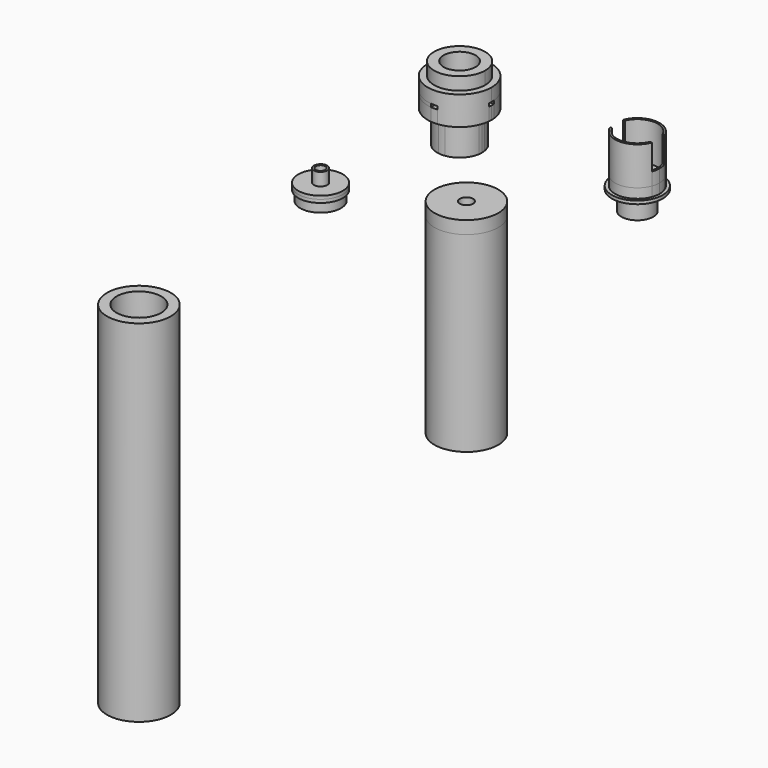
from build123d import *
from build123d import SkipClean  # not in build123d's __all__

# Parameters (mm, degrees)
F1_DEPTH  = 2
F2_DEPTH  = 7
F3_DEPTH  = 0.5
F5_DEPTH  = 2
F4_R      = 2.5
F6_DEPTH  = 4
F7_DEPTH  = 1
F8_R      = 2.5
F8_R_2    = 0.75
F9_DEPTH  = 2
F10_DEPTH = 5
F11_DEPTH = 2
F12_DEPTH = 6
F13_R     = 3.5
F13_R_2   = 3.2
F13_R_3   = 2.9
F14_DEPTH = 0.5
F15_DEPTH = 2
F13_R_4   = 1.05
F16_DEPTH = 0.5
F13_R_5   = 0.75
F17_DEPTH = 2.5
F18_R     = 5
F18_R_2   = 4
F19_DEPTH = 30
F18_R_3   = 1.35
F18_R_4   = 1.05
F20_DEPTH = 23
F21_DEPTH = 2
F22_R     = 4
F22_R_2   = 3.5
F23_DEPTH = 0.5
F24_R     = 5
F24_R_2   = 3.5
F25_DEPTH = 55
F26_DEPTH = 5


with BuildPart() as f1:
    # F0 (on Top) → F1 (new body)
    with BuildSketch(Plane.XY):
        with BuildLine():
            Line((-52.3957748821, 53.1159022585), (-50.8849393117, 53.1159022585))
            ThreePointArc((-50.8849393117, 53.1159022585), (-52.3243425913, 56.1514361644), (-55.3598764972, 57.590839444))
            Line((-55.3598764972, 57.590839444), (-55.3598764972, 56.0800038736))
            ThreePointArc((-55.3598764972, 56.0800038736), (-53.3850027631, 55.0907759926), (-52.3957748821, 53.1159022585))
        make_face()
        with BuildLine():
            Line((-59.3239781124, 53.1159022585), (-60.8348136828, 53.1159022585))
            ThreePointArc((-60.8348136828, 53.1159022585), (-60.8598764972, 52.6159022585), (-60.8348136828, 52.1159022585))
            Line((-60.8348136828, 52.1159022585), (-59.3239781124, 52.1159022585))
            ThreePointArc((-59.3239781124, 52.1159022585), (-59.3598764972, 52.6159022585), (-59.3239781124, 53.1159022585))
        make_face()
        with BuildLine():
            ThreePointArc((-56.3598764972, 47.6409650729), (-55.8598764972, 47.6159022585), (-55.3598764972, 47.6409650729))
            Line((-55.3598764972, 47.6409650729), (-55.3598764972, 49.1518006433))
            ThreePointArc((-55.3598764972, 49.1518006433), (-55.8598764972, 49.1159022585), (-56.3598764972, 49.1518006433))
            Line((-56.3598764972, 49.1518006433), (-56.3598764972, 47.6409650729))
        make_face()
        with BuildLine():
            ThreePointArc((-55.3598764972, 47.6409650729), (-52.3243425913, 49.0803683525), (-50.8849393117, 52.1159022585))
            Line((-50.8849393117, 52.1159022585), (-52.3957748821, 52.1159022585))
            ThreePointArc((-52.3957748821, 52.1159022585), (-53.3850027631, 50.1410285243), (-55.3598764972, 49.1518006433))
            Line((-55.3598764972, 49.1518006433), (-55.3598764972, 47.6409650729))
        make_face()
        with BuildLine():
            ThreePointArc((-52.3598764972, 52.6159022585), (-52.3688626292, 52.8665457773), (-52.3957748821, 53.1159022585))
            ThreePointArc((-52.3957748821, 53.1159022585), (-53.3850027631, 55.0907759926), (-55.3598764972, 56.0800038736))
            ThreePointArc((-55.3598764972, 56.0800038736), (-55.8598764972, 56.1159022585), (-56.3598764972, 56.0800038736))
            ThreePointArc((-56.3598764972, 56.0800038736), (-58.3347502314, 55.0907759926), (-59.3239781124, 53.1159022585))
            ThreePointArc((-59.3239781124, 53.1159022585), (-59.3598764972, 52.6159022585), (-59.3239781124, 52.1159022585))
            ThreePointArc((-59.3239781124, 52.1159022585), (-58.3347502314, 50.1410285243), (-56.3598764972, 49.1518006433))
            ThreePointArc((-56.3598764972, 49.1518006433), (-55.8598764972, 49.1159022585), (-55.3598764972, 49.1518006433))
            ThreePointArc((-55.3598764972, 49.1518006433), (-53.3850027631, 50.1410285243), (-52.3957748821, 52.1159022585))
            ThreePointArc((-52.3957748821, 52.1159022585), (-52.3688626292, 52.3652587397), (-52.3598764972, 52.6159022585))
        make_face()
        with BuildLine():
            ThreePointArc((-50.8849393117, 52.1159022585), (-50.8661461317, 52.3655883832), (-50.8598764972, 52.6159022585))
            ThreePointArc((-50.8598764972, 52.6159022585), (-50.8661461317, 52.8662161338), (-50.8849393117, 53.1159022585))
            Line((-50.8849393117, 53.1159022585), (-52.3957748821, 53.1159022585))
            ThreePointArc((-52.3957748821, 53.1159022585), (-52.3688626292, 52.8665457773), (-52.3598764972, 52.6159022585))
            ThreePointArc((-52.3598764972, 52.6159022585), (-52.3688626292, 52.3652587397), (-52.3957748821, 52.1159022585))
            Line((-52.3957748821, 52.1159022585), (-50.8849393117, 52.1159022585))
        make_face()
        with BuildLine():
            ThreePointArc((-60.8348136828, 52.1159022585), (-59.3954104032, 49.0803683525), (-56.3598764972, 47.6409650729))
            Line((-56.3598764972, 47.6409650729), (-56.3598764972, 49.1518006433))
            ThreePointArc((-56.3598764972, 49.1518006433), (-58.3347502314, 50.1410285243), (-59.3239781124, 52.1159022585))
            Line((-59.3239781124, 52.1159022585), (-60.8348136828, 52.1159022585))
        make_face()
        with BuildLine():
            Line((-55.3598764972, 56.0800038736), (-55.3598764972, 57.590839444))
            ThreePointArc((-55.3598764972, 57.590839444), (-55.8598764972, 57.6159022585), (-56.3598764972, 57.590839444))
            Line((-56.3598764972, 57.590839444), (-56.3598764972, 56.0800038736))
            ThreePointArc((-56.3598764972, 56.0800038736), (-55.8598764972, 56.1159022585), (-55.3598764972, 56.0800038736))
        make_face()
        with BuildLine():
            Line((-56.3598764972, 56.0800038736), (-56.3598764972, 57.590839444))
            ThreePointArc((-56.3598764972, 57.590839444), (-59.3954104032, 56.1514361644), (-60.8348136828, 53.1159022585))
            Line((-60.8348136828, 53.1159022585), (-59.3239781124, 53.1159022585))
            ThreePointArc((-59.3239781124, 53.1159022585), (-58.3347502314, 55.0907759926), (-56.3598764972, 56.0800038736))
        make_face()
    extrude(amount=-F1_DEPTH)

    # F0 (on Top) → F2 (join)
    with BuildSketch(Plane.XY):
        with BuildLine():
            ThreePointArc((-52.3598764972, 52.6159022585), (-52.3688626292, 52.8665457773), (-52.3957748821, 53.1159022585))
            ThreePointArc((-52.3957748821, 53.1159022585), (-53.3850027631, 55.0907759926), (-55.3598764972, 56.0800038736))
            ThreePointArc((-55.3598764972, 56.0800038736), (-55.8598764972, 56.1159022585), (-56.3598764972, 56.0800038736))
            ThreePointArc((-56.3598764972, 56.0800038736), (-58.3347502314, 55.0907759926), (-59.3239781124, 53.1159022585))
            ThreePointArc((-59.3239781124, 53.1159022585), (-59.3598764972, 52.6159022585), (-59.3239781124, 52.1159022585))
            ThreePointArc((-59.3239781124, 52.1159022585), (-58.3347502314, 50.1410285243), (-56.3598764972, 49.1518006433))
            ThreePointArc((-56.3598764972, 49.1518006433), (-55.8598764972, 49.1159022585), (-55.3598764972, 49.1518006433))
            ThreePointArc((-55.3598764972, 49.1518006433), (-53.3850027631, 50.1410285243), (-52.3957748821, 52.1159022585))
            ThreePointArc((-52.3957748821, 52.1159022585), (-52.3688626292, 52.3652587397), (-52.3598764972, 52.6159022585))
        make_face()
    extrude(amount=-F2_DEPTH)

    # F0 (on Top) → F3 (join)
    with BuildSketch(Plane.XY):
        with BuildLine():
            Line((-52.3957748821, 53.1159022585), (-50.8849393117, 53.1159022585))
            ThreePointArc((-50.8849393117, 53.1159022585), (-52.3243425913, 56.1514361644), (-55.3598764972, 57.590839444))
            Line((-55.3598764972, 57.590839444), (-55.3598764972, 56.0800038736))
            ThreePointArc((-55.3598764972, 56.0800038736), (-53.3850027631, 55.0907759926), (-52.3957748821, 53.1159022585))
        make_face()
        with BuildLine():
            ThreePointArc((-55.3598764972, 47.6409650729), (-52.3243425913, 49.0803683525), (-50.8849393117, 52.1159022585))
            Line((-50.8849393117, 52.1159022585), (-52.3957748821, 52.1159022585))
            ThreePointArc((-52.3957748821, 52.1159022585), (-53.3850027631, 50.1410285243), (-55.3598764972, 49.1518006433))
            Line((-55.3598764972, 49.1518006433), (-55.3598764972, 47.6409650729))
        make_face()
        with BuildLine():
            ThreePointArc((-60.8348136828, 52.1159022585), (-59.3954104032, 49.0803683525), (-56.3598764972, 47.6409650729))
            Line((-56.3598764972, 47.6409650729), (-56.3598764972, 49.1518006433))
            ThreePointArc((-56.3598764972, 49.1518006433), (-58.3347502314, 50.1410285243), (-59.3239781124, 52.1159022585))
            Line((-59.3239781124, 52.1159022585), (-60.8348136828, 52.1159022585))
        make_face()
        with BuildLine():
            Line((-56.3598764972, 56.0800038736), (-56.3598764972, 57.590839444))
            ThreePointArc((-56.3598764972, 57.590839444), (-59.3954104032, 56.1514361644), (-60.8348136828, 53.1159022585))
            Line((-60.8348136828, 53.1159022585), (-59.3239781124, 53.1159022585))
            ThreePointArc((-59.3239781124, 53.1159022585), (-58.3347502314, 55.0907759926), (-56.3598764972, 56.0800038736))
        make_face()
    extrude(amount=F3_DEPTH)

    # F4 (on face) → F5 (join)
    with BuildSketch(Plane.XY.offset(0.5)):
        with BuildLine():
            ThreePointArc((-60.8348136828, 53.1159022585), (-56.1101903725, 47.6221718929), (-50.8598764972, 52.6159022585))
            ThreePointArc((-50.8598764972, 52.6159022585), (-52.505774531, 56.324001502), (-56.3598764972, 57.590839444))
            Line((-56.3598764972, 57.590839444), (-56.3598764972, 56.5845292251))
            ThreePointArc((-56.3598764972, 56.5845292251), (-53.2141251862, 55.6159022585), (-51.8598764972, 52.6159022585))
            ThreePointArc((-51.8598764972, 52.6159022585), (-56.1103681474, 48.6237532215), (-59.8285034638, 53.1159022585))
            Line((-59.8285034638, 53.1159022585), (-60.8348136828, 53.1159022585))
        make_face()
        with BuildLine():
            Line((-56.3598764972, 56.5845292251), (-56.3598764972, 57.590839444))
            ThreePointArc((-56.3598764972, 57.590839444), (-59.3954104032, 56.1514361644), (-60.8348136828, 53.1159022585))
            Line((-60.8348136828, 53.1159022585), (-59.8285034638, 53.1159022585))
            ThreePointArc((-59.8285034638, 53.1159022585), (-58.688303622, 55.4443293832), (-56.3598764972, 56.5845292251))
        make_face()
        with BuildLine():
            Line((-56.3598764972, 56.0800038736), (-56.3598764972, 56.5845292251))
            ThreePointArc((-56.3598764972, 56.5845292251), (-58.688303622, 55.4443293832), (-59.8285034638, 53.1159022585))
            Line((-59.8285034638, 53.1159022585), (-59.3239781124, 53.1159022585))
            ThreePointArc((-59.3239781124, 53.1159022585), (-58.3347502314, 55.0907759926), (-56.3598764972, 56.0800038736))
        make_face()
    extrude(amount=F5_DEPTH)

    # F4 (on face) → F6 (join)
    with BuildSketch(Plane.XY.offset(0.5)):
        with BuildLine():
            Line((-56.3598764972, 56.0800038736), (-56.3598764972, 56.5845292251))
            ThreePointArc((-56.3598764972, 56.5845292251), (-58.688303622, 55.4443293832), (-59.8285034638, 53.1159022585))
            Line((-59.8285034638, 53.1159022585), (-59.3239781124, 53.1159022585))
            ThreePointArc((-59.3239781124, 53.1159022585), (-58.3347502314, 55.0907759926), (-56.3598764972, 56.0800038736))
        make_face()
        with BuildLine():
            ThreePointArc((-51.8598764972, 52.6159022585), (-53.2141251862, 55.6159022585), (-56.3598764972, 56.5845292251))
            Line((-56.3598764972, 56.5845292251), (-56.3598764972, 56.0800038736))
            ThreePointArc((-56.3598764972, 56.0800038736), (-58.3347502314, 55.0907759926), (-59.3239781124, 53.1159022585))
            Line((-59.3239781124, 53.1159022585), (-59.8285034638, 53.1159022585))
            ThreePointArc((-59.8285034638, 53.1159022585), (-56.1103681474, 48.6237532215), (-51.8598764972, 52.6159022585))
        make_face()
        with Locations((-55.8598764972, 52.6159022585)):
            Circle(F4_R, mode=Mode.SUBTRACT)
    extrude(amount=F6_DEPTH)

    # F0 (on Top) → F7 (cut)
    with BuildSketch(Plane.XY):
        with BuildLine():
            ThreePointArc((-52.3598764972, 52.6159022585), (-52.3688626292, 52.8665457773), (-52.3957748821, 53.1159022585))
            ThreePointArc((-52.3957748821, 53.1159022585), (-53.3850027631, 55.0907759926), (-55.3598764972, 56.0800038736))
            ThreePointArc((-55.3598764972, 56.0800038736), (-55.8598764972, 56.1159022585), (-56.3598764972, 56.0800038736))
            ThreePointArc((-56.3598764972, 56.0800038736), (-58.3347502314, 55.0907759926), (-59.3239781124, 53.1159022585))
            ThreePointArc((-59.3239781124, 53.1159022585), (-59.3598764972, 52.6159022585), (-59.3239781124, 52.1159022585))
            ThreePointArc((-59.3239781124, 52.1159022585), (-58.3347502314, 50.1410285243), (-56.3598764972, 49.1518006433))
            ThreePointArc((-56.3598764972, 49.1518006433), (-55.8598764972, 49.1159022585), (-55.3598764972, 49.1518006433))
            ThreePointArc((-55.3598764972, 49.1518006433), (-53.3850027631, 50.1410285243), (-52.3957748821, 52.1159022585))
            ThreePointArc((-52.3957748821, 52.1159022585), (-52.3688626292, 52.3652587397), (-52.3598764972, 52.6159022585))
        make_face()
    extrude(amount=-F7_DEPTH, mode=Mode.SUBTRACT)


with BuildPart() as f9:
    # F8 (on Top) → F9 (new body)
    with BuildSketch(Plane.XY):
        with BuildLine():
            Line((-22.5184842519, 50.6979984153), (-22.1950697086, 50.6979984153))
            ThreePointArc((-22.1950697086, 50.6979984153), (-25.4642439163, 52.9479984153), (-28.7334181239, 50.6979984153))
            Line((-28.7334181239, 50.6979984153), (-28.4100035806, 50.6979984153))
            ThreePointArc((-28.4100035806, 50.6979984153), (-25.4642439163, 52.6479984153), (-22.5184842519, 50.6979984153))
        make_face()
        with BuildLine():
            Line((-28.4100035806, 50.6979984153), (-28.7334181239, 50.6979984153))
            ThreePointArc((-28.7334181239, 50.6979984153), (-28.9642439163, 49.4479984153), (-28.7334181239, 48.1979984153))
            Line((-28.7334181239, 48.1979984153), (-28.4100035806, 48.1979984153))
            ThreePointArc((-28.4100035806, 48.1979984153), (-28.6642439163, 49.4479984153), (-28.4100035806, 50.6979984153))
        make_face()
        with BuildLine():
            ThreePointArc((-28.7334181239, 48.1979984153), (-25.4642439163, 45.9479984153), (-22.1950697086, 48.1979984153))
            Line((-22.1950697086, 48.1979984153), (-22.5184842519, 48.1979984153))
            ThreePointArc((-22.5184842519, 48.1979984153), (-25.4642439163, 46.2479984153), (-28.4100035806, 48.1979984153))
            Line((-28.4100035806, 48.1979984153), (-28.7334181239, 48.1979984153))
        make_face()
        with BuildLine():
            ThreePointArc((-22.1950697086, 48.1979984153), (-22.0224340924, 48.8124316315), (-21.9642439163, 49.4479984153))
            ThreePointArc((-21.9642439163, 49.4479984153), (-22.0224340924, 50.083565199), (-22.1950697086, 50.6979984153))
            Line((-22.1950697086, 50.6979984153), (-22.5184842519, 50.6979984153))
            ThreePointArc((-22.5184842519, 50.6979984153), (-22.3284480902, 50.085795042), (-22.2642439163, 49.4479984153))
            ThreePointArc((-22.2642439163, 49.4479984153), (-22.3284480902, 48.8102017886), (-22.5184842519, 48.1979984153))
            Line((-22.5184842519, 48.1979984153), (-22.1950697086, 48.1979984153))
        make_face()
        with BuildLine():
            ThreePointArc((-22.2642439163, 49.4479984153), (-22.3284480902, 50.085795042), (-22.5184842519, 50.6979984153))
            ThreePointArc((-22.5184842519, 50.6979984153), (-25.4642439163, 52.6479984153), (-28.4100035806, 50.6979984153))
            ThreePointArc((-28.4100035806, 50.6979984153), (-28.6642439163, 49.4479984153), (-28.4100035806, 48.1979984153))
            ThreePointArc((-28.4100035806, 48.1979984153), (-25.4642439163, 46.2479984153), (-22.5184842519, 48.1979984153))
            ThreePointArc((-22.5184842519, 48.1979984153), (-22.3284480902, 48.8102017886), (-22.2642439163, 49.4479984153))
        make_face()
        with Locations((-25.4642439163, 49.4479984153)):
            Circle(F8_R, mode=Mode.SUBTRACT)
        with Locations((-25.4642439163, 49.4479984153)):
            Circle(F8_R)
        with Locations((-25.4642439163, 49.4479984153)):
            Circle(F8_R_2, mode=Mode.SUBTRACT)
    extrude(amount=-F9_DEPTH)

    # F8 (on Top) → F10 (join)
    with BuildSketch(Plane.XY):
        with Locations((-25.4642439163, 49.4479984153)):
            Circle(F8_R)
        with Locations((-25.4642439163, 49.4479984153)):
            Circle(F8_R_2, mode=Mode.SUBTRACT)
    extrude(amount=-F10_DEPTH)

    # F8 (on Top) → F11 (join)
    with BuildSketch(Plane.XY):
        with BuildLine():
            ThreePointArc((-22.1950697086, 48.1979984153), (-22.0224340924, 48.8124316315), (-21.9642439163, 49.4479984153))
            ThreePointArc((-21.9642439163, 49.4479984153), (-22.0224340924, 50.083565199), (-22.1950697086, 50.6979984153))
            Line((-22.1950697086, 50.6979984153), (-22.5184842519, 50.6979984153))
            ThreePointArc((-22.5184842519, 50.6979984153), (-22.3284480902, 50.085795042), (-22.2642439163, 49.4479984153))
            ThreePointArc((-22.2642439163, 49.4479984153), (-22.3284480902, 48.8102017886), (-22.5184842519, 48.1979984153))
            Line((-22.5184842519, 48.1979984153), (-22.1950697086, 48.1979984153))
        make_face()
        with BuildLine():
            Line((-28.4100035806, 50.6979984153), (-28.7334181239, 50.6979984153))
            ThreePointArc((-28.7334181239, 50.6979984153), (-28.9642439163, 49.4479984153), (-28.7334181239, 48.1979984153))
            Line((-28.7334181239, 48.1979984153), (-28.4100035806, 48.1979984153))
            ThreePointArc((-28.4100035806, 48.1979984153), (-28.6642439163, 49.4479984153), (-28.4100035806, 50.6979984153))
        make_face()
    extrude(amount=F11_DEPTH)

    # F8 (on Top) → F12 (join)
    with BuildSketch(Plane.XY):
        with BuildLine():
            ThreePointArc((-28.7334181239, 48.1979984153), (-25.4642439163, 45.9479984153), (-22.1950697086, 48.1979984153))
            Line((-22.1950697086, 48.1979984153), (-22.5184842519, 48.1979984153))
            ThreePointArc((-22.5184842519, 48.1979984153), (-25.4642439163, 46.2479984153), (-28.4100035806, 48.1979984153))
            Line((-28.4100035806, 48.1979984153), (-28.7334181239, 48.1979984153))
        make_face()
        with BuildLine():
            Line((-22.5184842519, 50.6979984153), (-22.1950697086, 50.6979984153))
            ThreePointArc((-22.1950697086, 50.6979984153), (-25.4642439163, 52.9479984153), (-28.7334181239, 50.6979984153))
            Line((-28.7334181239, 50.6979984153), (-28.4100035806, 50.6979984153))
            ThreePointArc((-28.4100035806, 50.6979984153), (-25.4642439163, 52.6479984153), (-22.5184842519, 50.6979984153))
        make_face()
    with SkipClean():  # cleaning this boolean's faces spoils the solid; the shape is the same uncleaned
        extrude(amount=F12_DEPTH)


with BuildPart() as f14:
    # F13 (on Top) → F14 (new body)
    with BuildSketch(Plane.XY):
        with Locations((-53.8438744843, 22.8516831994)):
            Circle(F13_R)
        with Locations((-53.8438744843, 22.8516831994)):
            Circle(F13_R_2, mode=Mode.SUBTRACT)
        with Locations((-53.8438744843, 22.8516831994)):
            Circle(F13_R_2)
        with Locations((-53.8438744843, 22.8516831994)):
            Circle(F13_R_3, mode=Mode.SUBTRACT)
    extrude(amount=-F14_DEPTH)

    # F13 (on Top) → F15 (join)
    with BuildSketch(Plane.XY):
        with Locations((-53.8438744843, 22.8516831994)):
            Circle(F13_R_2)
        with Locations((-53.8438744843, 22.8516831994)):
            Circle(F13_R_3, mode=Mode.SUBTRACT)
    extrude(amount=-F15_DEPTH)

    # F13 (on Top) → F16 (join)
    with BuildSketch(Plane.XY):
        with Locations((-53.8438744843, 22.8516831994)):
            Circle(F13_R)
        with Locations((-53.8438744843, 22.8516831994)):
            Circle(F13_R_2, mode=Mode.SUBTRACT)
        with Locations((-53.8438744843, 22.8516831994)):
            Circle(F13_R_2)
        with Locations((-53.8438744843, 22.8516831994)):
            Circle(F13_R_3, mode=Mode.SUBTRACT)
        with Locations((-53.8438744843, 22.8516831994)):
            Circle(F13_R_3)
        with Locations((-53.8438744843, 22.8516831994)):
            Circle(F13_R_4, mode=Mode.SUBTRACT)
    extrude(amount=F16_DEPTH)

    # F13 (on Top) → F17 (join)
    with BuildSketch(Plane.XY):
        with Locations((-53.8438744843, 22.8516831994)):
            Circle(F13_R_4)
        with Locations((-53.8438744843, 22.8516831994)):
            Circle(F13_R_5, mode=Mode.SUBTRACT)
    extrude(amount=F17_DEPTH)


with BuildPart() as f19:
    # F18 (on Top) → F19 (new body)
    with BuildSketch(Plane.XY):
        with Locations((-35.0039340556, 27.8797037899)):
            Circle(F18_R)
        with Locations((-35.0039340556, 27.8797037899)):
            Circle(F18_R_2, mode=Mode.SUBTRACT)
    extrude(amount=-F19_DEPTH)


with BuildPart() as f20:
    # F18 (on Top) → F20 (new body)
    with BuildSketch(Plane.XY):
        with Locations((-35.0039340556, 27.8797037899)):
            Circle(F18_R_3)
        with Locations((-35.0039340556, 27.8797037899)):
            Circle(F18_R_4, mode=Mode.SUBTRACT)
    extrude(amount=-F20_DEPTH)


with BuildPart() as f21:
    # F18 (on Top) → F21 (new body)
    with BuildSketch(Plane.XY):
        with Locations((-35.0039340556, 27.8797037899)):
            Circle(F18_R)
        with Locations((-35.0039340556, 27.8797037899)):
            Circle(F18_R_2, mode=Mode.SUBTRACT)
        with Locations((-35.0039340556, 27.8797037899)):
            Circle(F18_R_2)
        with Locations((-35.0039340556, 27.8797037899)):
            Circle(F18_R_3, mode=Mode.SUBTRACT)
        with Locations((-35.0039340556, 27.8797037899)):
            Circle(F18_R_3)
        with Locations((-35.0039340556, 27.8797037899)):
            Circle(F18_R_4, mode=Mode.SUBTRACT)
    extrude(amount=F21_DEPTH)


with BuildPart() as f23:
    # F22 (on face) → F23 (new body)
    with BuildSketch(Plane(origin=(0, 0, -2), x_dir=(1, 0, 0), z_dir=(0, 0, -1))):
        with Locations((-25.4642439163, -49.4479984153)):
            Circle(F22_R)
        with Locations((-25.4642439163, -49.4479984153)):
            Circle(F22_R_2, mode=Mode.SUBTRACT)
    extrude(amount=-F23_DEPTH)


with BuildPart() as f25:
    # F24 (on Top) → F25 (new body)
    with BuildSketch(Plane.XY):
        with Locations((-51.6030266881, -15.5521593988)):
            Circle(F24_R)
        with Locations((-51.6030266881, -15.5521593988)):
            Circle(F24_R_2, mode=Mode.SUBTRACT)
        with Locations((-51.6030266881, -15.5521593988)):
            Circle(F24_R_2)
    extrude(amount=-F25_DEPTH)

    # F24 (on Top) → F26 (cut)
    with BuildSketch(Plane.XY):
        with Locations((-51.6030266881, -15.5521593988)):
            Circle(F24_R_2)
    extrude(amount=-F26_DEPTH, mode=Mode.SUBTRACT)


solid = Compound([f1.part, f9.part, f14.part, f19.part, f20.part, f21.part, f23.part, f25.part])
